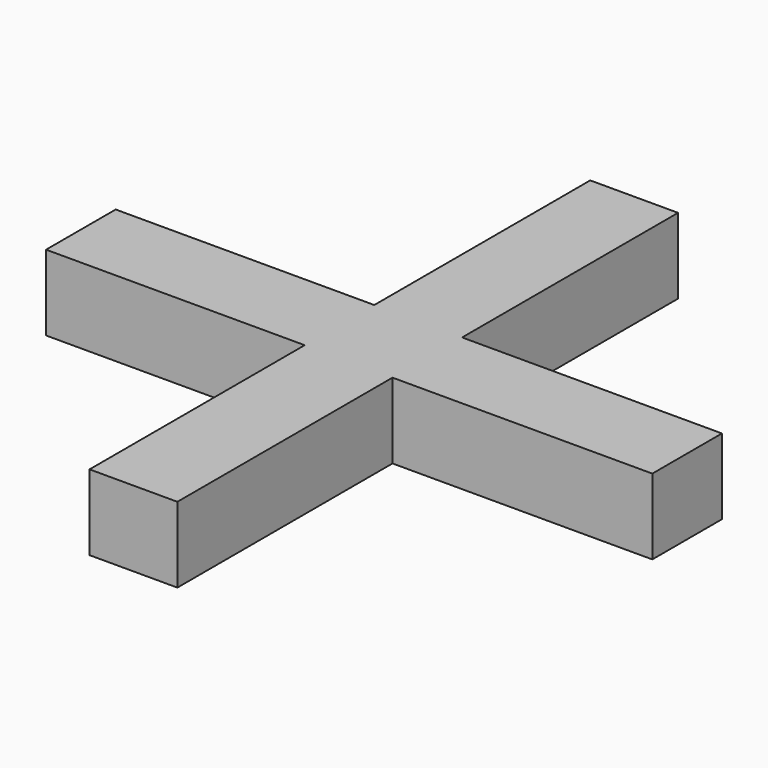
from build123d import *

# Parameters (mm, degrees)
F0_TEXT_SIZE = 0.5984504408
F1_DEPTH     = 0.035


# Not quite as in the source:
# - Text() gives the source's letters only with a copy of the font that has no kerning and outlines rounded to 1/6400 em; it was checked with that copy


with BuildPart() as f1:
    # F0 (on Top) → F1 (new body)
    with BuildSketch(Plane.XY):
        with Locations((-0.175, -0.2153843174)):
            Text('+', F0_TEXT_SIZE, font='Open Sans', text_align=(TextAlign.LEFT, TextAlign.BOTTOM))
    extrude(amount=F1_DEPTH)


solid = f1.part
